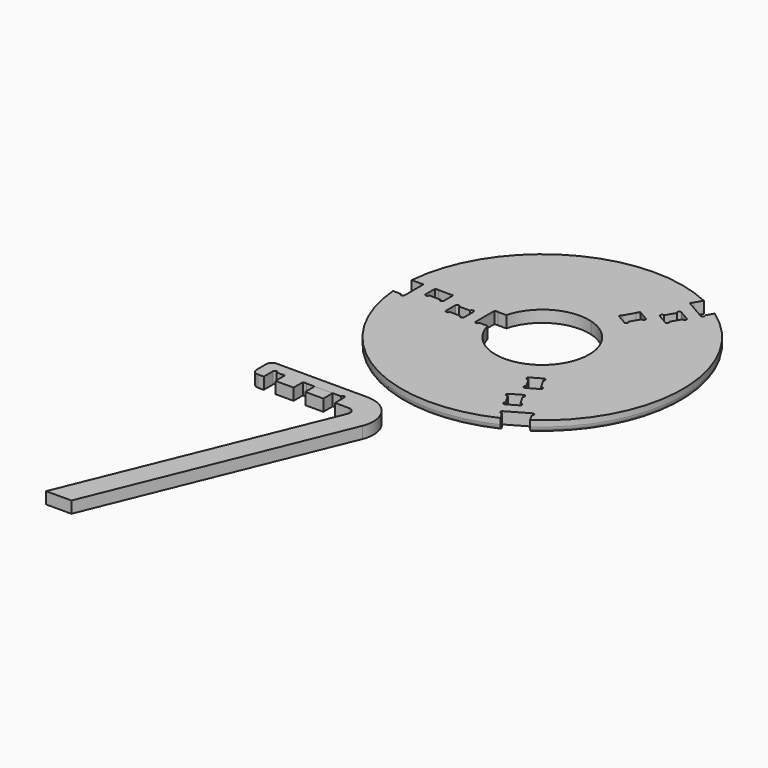
from build123d import *

# Parameters (mm, degrees)
F3_DEPTH = 25.4
F4_DEPTH = 25.4
F5_W     = 39.1830229406
F5_H     = 25.4
F6_DEPTH = 25.4
F7_DEPTH = 25.4
F8_R     = 12.7
F9_R     = 12.7
F10_R    = 12.7
F11_R    = 12.7


# Not quite as in the source:
# - a feature names something its author has since deleted; it is built from what else it names


with BuildPart() as f3:
    # F1 (on Top) → F3 (new body)
    with BuildSketch(Plane.XY):
        with BuildLine():
            Line((27.1898432407, 97.8941899427), (129.8728661813, 275.7464027505))
            ThreePointArc((129.8728661813, 275.7464027505), (-152.4, 263.9645430735), (-303.7398228748, 25.4))
            Line((-303.7398228748, 25.4), (-98.3737769937, 25.4))
            ThreePointArc((-98.3737769937, 25.4), (-50.8, 87.9881810245), (27.1898432407, 97.8941899427))
        make_face()
    extrude(amount=F3_DEPTH)

    # F10
    f10_edges = [f3.edges().sort_by_distance(p)[0] for p in [
        (-152.4, 263.964543, 25.4),
    ]]
    fillet(f10_edges, radius=F10_R)


with BuildPart() as f4:
    # F2 (on face) → F4 (new body)
    with BuildSketch(Plane.XY):
        with BuildLine():
            Line((-285.9598228748, -25.4), (-303.7398228748, -25.4))
            ThreePointArc((-303.7398228748, -25.4), (-152.4, -263.9645430735), (129.8728661813, -275.7464027505))
            Line((129.8728661813, -275.7464027505), (120.9828661813, -260.3484710713))
            ThreePointArc((120.9828661813, -260.3484710713), (115.7783093928, -258.9539142828), (117.1728661813, -253.7493574944))
            Line((117.1728661813, -253.7493574944), (104.4728661813, -231.7523122383))
            ThreePointArc((104.4728661813, -231.7523122383), (99.2683093928, -230.3577554499), (100.6628661813, -225.1531986615))
            Line((100.6628661813, -225.1531986615), (88.691354711, -204.4179325515))
            ThreePointArc((88.691354711, -204.4179325515), (83.4867979226, -203.0233757631), (84.881354711, -197.8188189747))
            Line((84.881354711, -197.8188189747), (27.1898432407, -97.8941899427))
            ThreePointArc((27.1898432407, -97.8941899427), (-50.8, -87.9881810245), (-98.3737769937, -25.4))
            Line((-98.3737769937, -25.4), (-116.1537769937, -25.4))
            ThreePointArc((-116.1537769937, -25.4), (-119.9637769937, -29.21), (-123.7737769937, -25.4))
            Line((-123.7737769937, -25.4), (-149.1737769937, -25.4))
            ThreePointArc((-149.1737769937, -25.4), (-152.9837769937, -29.21), (-156.7937769937, -25.4))
            Line((-156.7937769937, -25.4), (-180.7367999342, -25.4))
            ThreePointArc((-180.7367999342, -25.4), (-184.5467999342, -29.21), (-188.3567999342, -25.4))
            Line((-188.3567999342, -25.4), (-278.3398228748, -25.4))
            ThreePointArc((-278.3398228748, -25.4), (-282.1498228748, -29.21), (-285.9598228748, -25.4))
        make_face()
        with BuildLine():
            ThreePointArc((304.8, 0), (270.0904370763, 141.2593211081), (173.8669566935, 250.3464027505))
            Line((173.8669566935, 250.3464027505), (164.9769566935, 234.9484710713))
            ThreePointArc((164.9769566935, 234.9484710713), (166.3715134819, 229.7439142828), (161.1669566935, 228.3493574944))
            Line((161.1669566935, 228.3493574944), (148.4669566935, 206.3523122383))
            ThreePointArc((148.4669566935, 206.3523122383), (149.8615134819, 201.1477554499), (144.6569566935, 199.7531986615))
            Line((144.6569566935, 199.7531986615), (132.6854452232, 179.0179325515))
            ThreePointArc((132.6854452232, 179.0179325515), (134.0800020117, 173.8133757631), (128.8754452232, 172.4188189747))
            Line((128.8754452232, 172.4188189747), (71.183933753, 72.4941899427))
            ThreePointArc((71.183933753, 72.4941899427), (93.687906555, 39.3082200735), (101.6, 0))
            ThreePointArc((101.6, 0), (93.687906555, -39.3082200735), (71.183933753, -72.4941899427))
            Line((71.183933753, -72.4941899427), (96.583933753, -116.488280455))
            ThreePointArc((96.583933753, -116.488280455), (101.7884905414, -117.8828372434), (100.393933753, -123.0873940318))
            Line((100.393933753, -123.0873940318), (112.3654452232, -143.8226601417))
            ThreePointArc((112.3654452232, -143.8226601417), (117.5700020117, -145.2172169302), (116.1754452232, -150.4217737186))
            Line((116.1754452232, -150.4217737186), (161.1669566935, -228.3493574944))
            ThreePointArc((161.1669566935, -228.3493574944), (166.3715134819, -229.7439142828), (164.9769566935, -234.9484710713))
            Line((164.9769566935, -234.9484710713), (173.8669566935, -250.3464027505))
            ThreePointArc((173.8669566935, -250.3464027505), (270.0904370763, -141.2593211081), (304.8, 0))
        make_face()
        with BuildLine():
            ThreePointArc((129.8728661813, 275.7464027505), (-152.4, 263.9645430735), (-303.7398228748, 25.4))
            Line((-303.7398228748, 25.4), (-285.9598228748, 25.4))
            ThreePointArc((-285.9598228748, 25.4), (-282.1498228748, 29.21), (-278.3398228748, 25.4))
            Line((-278.3398228748, 25.4), (-252.9398228748, 25.4))
            ThreePointArc((-252.9398228748, 25.4), (-249.1298228748, 29.21), (-245.3198228748, 25.4))
            Line((-245.3198228748, 25.4), (-221.3767999342, 25.4))
            ThreePointArc((-221.3767999342, 25.4), (-217.5667999342, 29.21), (-213.7567999342, 25.4))
            Line((-213.7567999342, 25.4), (-123.7737769937, 25.4))
            ThreePointArc((-123.7737769937, 25.4), (-119.9637769937, 29.21), (-116.1537769937, 25.4))
            Line((-116.1537769937, 25.4), (-98.3737769937, 25.4))
            ThreePointArc((-98.3737769937, 25.4), (-50.8, 87.9881810245), (27.1898432407, 97.8941899427))
            Line((27.1898432407, 97.8941899427), (52.5898432407, 141.888280455))
            ThreePointArc((52.5898432407, 141.888280455), (51.1952864523, 147.0928372434), (56.3998432407, 148.4873940318))
            Line((56.3998432407, 148.4873940318), (68.371354711, 169.2226601417))
            ThreePointArc((68.371354711, 169.2226601417), (66.9767979226, 174.4272169302), (72.181354711, 175.8217737186))
            Line((72.181354711, 175.8217737186), (117.1728661813, 253.7493574944))
            ThreePointArc((117.1728661813, 253.7493574944), (115.7783093928, 258.9539142828), (120.9828661813, 260.3484710713))
            Line((120.9828661813, 260.3484710713), (129.8728661813, 275.7464027505))
        make_face()
        with BuildLine():
            Line((-252.9398228748, 25.4), (-278.3398228748, 25.4))
            Line((-278.3398228748, 25.4), (-278.3398228748, -25.4))
            Line((-278.3398228748, -25.4), (-188.3567999342, -25.4))
            Line((-188.3567999342, -25.4), (-188.3567999342, 0))
            ThreePointArc((-188.3567999342, 0), (-184.5467999342, 3.81), (-180.7367999342, 0))
            Line((-180.7367999342, 0), (-156.7937769937, 0))
            ThreePointArc((-156.7937769937, 0), (-152.9837769937, 3.81), (-149.1737769937, 0))
            Line((-149.1737769937, 0), (-149.1737769937, -25.4))
            Line((-149.1737769937, -25.4), (-123.7737769937, -25.4))
            Line((-123.7737769937, -25.4), (-123.7737769937, 25.4))
            Line((-123.7737769937, 25.4), (-213.7567999342, 25.4))
            Line((-213.7567999342, 25.4), (-213.7567999342, 0))
            ThreePointArc((-213.7567999342, 0), (-217.5667999342, -3.81), (-221.3767999342, 0))
            Line((-221.3767999342, 0), (-245.3198228748, 0))
            ThreePointArc((-245.3198228748, 0), (-249.1298228748, -3.81), (-252.9398228748, 0))
            Line((-252.9398228748, 0), (-252.9398228748, 25.4))
        make_face()
        with BuildLine():
            Line((161.1669566935, 228.3493574944), (117.1728661813, 253.7493574944))
            Line((117.1728661813, 253.7493574944), (72.181354711, 175.8217737186))
            Line((72.181354711, 175.8217737186), (94.1783999671, 163.1217737186))
            ThreePointArc((94.1783999671, 163.1217737186), (95.5729567555, 157.9172169302), (90.3683999671, 156.5226601417))
            Line((90.3683999671, 156.5226601417), (78.3968884968, 135.7873940318))
            ThreePointArc((78.3968884968, 135.7873940318), (79.7914452853, 130.5828372434), (74.5868884968, 129.188280455))
            Line((74.5868884968, 129.188280455), (52.5898432407, 141.888280455))
            Line((52.5898432407, 141.888280455), (27.1898432407, 97.8941899427))
            ThreePointArc((27.1898432407, 97.8941899427), (50.8, 87.9881810245), (71.183933753, 72.4941899427))
            Line((71.183933753, 72.4941899427), (128.8754452232, 172.4188189747))
            Line((128.8754452232, 172.4188189747), (106.8783999671, 185.1188189747))
            ThreePointArc((106.8783999671, 185.1188189747), (105.4838431787, 190.3233757631), (110.6883999671, 191.7179325515))
            Line((110.6883999671, 191.7179325515), (122.6599114374, 212.4531986615))
            ThreePointArc((122.6599114374, 212.4531986615), (121.265354649, 217.6577554499), (126.4699114374, 219.0523122383))
            Line((126.4699114374, 219.0523122383), (148.4669566935, 206.3523122383))
            Line((148.4669566935, 206.3523122383), (161.1669566935, 228.3493574944))
        make_face()
        with BuildLine():
            Line((104.4728661813, -231.7523122383), (117.1728661813, -253.7493574944))
            Line((117.1728661813, -253.7493574944), (161.1669566935, -228.3493574944))
            Line((161.1669566935, -228.3493574944), (116.1754452232, -150.4217737186))
            Line((116.1754452232, -150.4217737186), (94.1783999671, -163.1217737186))
            ThreePointArc((94.1783999671, -163.1217737186), (88.9738431787, -161.7272169302), (90.3683999671, -156.5226601417))
            Line((90.3683999671, -156.5226601417), (78.3968884968, -135.7873940318))
            ThreePointArc((78.3968884968, -135.7873940318), (73.1923317084, -134.3928372434), (74.5868884968, -129.188280455))
            Line((74.5868884968, -129.188280455), (96.583933753, -116.488280455))
            Line((96.583933753, -116.488280455), (71.183933753, -72.4941899427))
            ThreePointArc((71.183933753, -72.4941899427), (50.8, -87.9881810245), (27.1898432407, -97.8941899427))
            Line((27.1898432407, -97.8941899427), (84.881354711, -197.8188189747))
            Line((84.881354711, -197.8188189747), (106.8783999671, -185.1188189747))
            ThreePointArc((106.8783999671, -185.1188189747), (112.0829567555, -186.5133757631), (110.6883999671, -191.7179325515))
            Line((110.6883999671, -191.7179325515), (122.6599114374, -212.4531986615))
            ThreePointArc((122.6599114374, -212.4531986615), (127.8644682258, -213.8477554499), (126.4699114374, -219.0523122383))
            Line((126.4699114374, -219.0523122383), (104.4728661813, -231.7523122383))
        make_face()
    extrude(amount=F4_DEPTH)

    # F11
    f11_edges = [f4.edges().sort_by_distance(p)[0] for p in [
        (-152.4, 263.964543, 0),
        (-152.4, -263.964543, 0),
        (304.8, 0, 0),
    ]]
    fillet(f11_edges, radius=F11_R)


with BuildPart() as f6:
    # F5 (on face) → F6 (new body)
    with BuildSketch(Plane.XY):
        with BuildLine():
            Line((-93.7748046815, -356.7161729336), (-303.7398228748, -356.7161729336))
            Line((-303.7398228748, -356.7161729336), (-303.7398228748, -407.5161729336))
            Line((-303.7398228748, -407.5161729336), (-278.3398228748, -407.5161729336))
            Line((-278.3398228748, -407.5161729336), (-278.3398228748, -382.1161729336))
            ThreePointArc((-278.3398228748, -382.1161729336), (-274.5298228748, -378.3061729336), (-270.7198228748, -382.1161729336))
            Line((-270.7198228748, -382.1161729336), (-260.5598228748, -382.1161729336))
            ThreePointArc((-260.5598228748, -382.1161729336), (-256.7498228748, -378.3061729336), (-252.9398228748, -382.1161729336))
            Line((-252.9398228748, -382.1161729336), (-213.7567999342, -382.1161729336))
            ThreePointArc((-213.7567999342, -382.1161729336), (-209.9467999342, -378.3061729336), (-206.1367999342, -382.1161729336))
            Line((-206.1367999342, -382.1161729336), (-195.9767999342, -382.1161729336))
            ThreePointArc((-195.9767999342, -382.1161729336), (-192.1667999342, -378.3061729336), (-188.3567999342, -382.1161729336))
            Line((-188.3567999342, -382.1161729336), (-149.1737769937, -382.1161729336))
            ThreePointArc((-149.1737769937, -382.1161729336), (-145.3637769937, -378.3061729336), (-141.5537769937, -382.1161729336))
            Line((-141.5537769937, -382.1161729336), (-131.3937769937, -382.1161729336))
            ThreePointArc((-131.3937769937, -382.1161729336), (-127.5837769937, -378.3061729336), (-123.7737769937, -382.1161729336))
            Line((-123.7737769937, -382.1161729336), (-123.7737769937, -407.5161729336))
            Line((-123.7737769937, -407.5161729336), (-93.7748046815, -407.5161729336))
            ThreePointArc((-93.7748046815, -407.5161729336), (-83.2290397207, -413.1396737009), (-82.0225058384, -425.0300561792))
            Line((-82.0225058384, -425.0300561792), (-303.7398228748, -966.3161729336))
            Line((-303.7398228748, -966.3161729336), (-248.8433291239, -966.3161729336))
            Line((-248.8433291239, -966.3161729336), (-35.0133104659, -444.2855891614))
            ThreePointArc((-35.0133104659, -444.2855891614), (-41.0459798773, -384.83367677), (-93.7748046815, -356.7161729336))
        make_face()
        with Locations((-168.7652884639, -394.8161729336)):
            Rectangle(F5_W, F5_H)
        with BuildLine():
            Line((-260.5598228748, -382.1161729336), (-252.9398228748, -382.1161729336))
            ThreePointArc((-252.9398228748, -382.1161729336), (-256.7498228748, -378.3061729336), (-260.5598228748, -382.1161729336))
        make_face()
        with BuildLine():
            ThreePointArc((-206.1367999342, -382.1161729336), (-209.9467999342, -378.3061729336), (-213.7567999342, -382.1161729336))
            Line((-213.7567999342, -382.1161729336), (-206.1367999342, -382.1161729336))
        make_face()
    extrude(amount=F6_DEPTH)

    # F8
    f8_edges = [f6.edges().sort_by_distance(p)[0] for p in [
        (-303.739823, -356.716173, 12.7),
        (-303.739823, -407.516173, 12.7),
    ]]
    fillet(f8_edges, radius=F8_R)


with BuildPart() as f7:
    # F5 (on face) → F7 (new body)
    with BuildSketch(Plane.XY):
        with BuildLine():
            Line((-93.7748046815, -356.7161729336), (-303.7398228748, -356.7161729336))
            Line((-303.7398228748, -356.7161729336), (-303.7398228748, -407.5161729336))
            Line((-303.7398228748, -407.5161729336), (-278.3398228748, -407.5161729336))
            Line((-278.3398228748, -407.5161729336), (-278.3398228748, -382.1161729336))
            ThreePointArc((-278.3398228748, -382.1161729336), (-274.5298228748, -378.3061729336), (-270.7198228748, -382.1161729336))
            Line((-270.7198228748, -382.1161729336), (-260.5598228748, -382.1161729336))
            ThreePointArc((-260.5598228748, -382.1161729336), (-256.7498228748, -378.3061729336), (-252.9398228748, -382.1161729336))
            Line((-252.9398228748, -382.1161729336), (-213.7567999342, -382.1161729336))
            ThreePointArc((-213.7567999342, -382.1161729336), (-209.9467999342, -378.3061729336), (-206.1367999342, -382.1161729336))
            Line((-206.1367999342, -382.1161729336), (-195.9767999342, -382.1161729336))
            ThreePointArc((-195.9767999342, -382.1161729336), (-192.1667999342, -378.3061729336), (-188.3567999342, -382.1161729336))
            Line((-188.3567999342, -382.1161729336), (-149.1737769937, -382.1161729336))
            ThreePointArc((-149.1737769937, -382.1161729336), (-145.3637769937, -378.3061729336), (-141.5537769937, -382.1161729336))
            Line((-141.5537769937, -382.1161729336), (-131.3937769937, -382.1161729336))
            ThreePointArc((-131.3937769937, -382.1161729336), (-127.5837769937, -378.3061729336), (-123.7737769937, -382.1161729336))
            Line((-123.7737769937, -382.1161729336), (-123.7737769937, -407.5161729336))
            Line((-123.7737769937, -407.5161729336), (-93.7748046815, -407.5161729336))
            ThreePointArc((-93.7748046815, -407.5161729336), (-83.2290397207, -413.1396737009), (-82.0225058384, -425.0300561792))
            Line((-82.0225058384, -425.0300561792), (-303.7398228748, -966.3161729336))
            Line((-303.7398228748, -966.3161729336), (-248.8433291239, -966.3161729336))
            Line((-248.8433291239, -966.3161729336), (-35.0133104659, -444.2855891614))
            ThreePointArc((-35.0133104659, -444.2855891614), (-41.0459798773, -384.83367677), (-93.7748046815, -356.7161729336))
        make_face()
        with Locations((-233.3483114045, -394.8161729336)):
            Rectangle(F5_W, F5_H)
        with BuildLine():
            Line((-195.9767999342, -382.1161729336), (-188.3567999342, -382.1161729336))
            ThreePointArc((-188.3567999342, -382.1161729336), (-192.1667999342, -378.3061729336), (-195.9767999342, -382.1161729336))
        make_face()
        with BuildLine():
            ThreePointArc((-141.5537769937, -382.1161729336), (-145.3637769937, -378.3061729336), (-149.1737769937, -382.1161729336))
            Line((-149.1737769937, -382.1161729336), (-141.5537769937, -382.1161729336))
        make_face()
    extrude(amount=F7_DEPTH)

    # F9
    f9_edges = [f7.edges().sort_by_distance(p)[0] for p in [
        (-303.739823, -356.716173, 12.7),
        (-303.739823, -407.516173, 12.7),
    ]]
    fillet(f9_edges, radius=F9_R)


solid = Compound([f3.part, f4.part, f6.part, f7.part])
